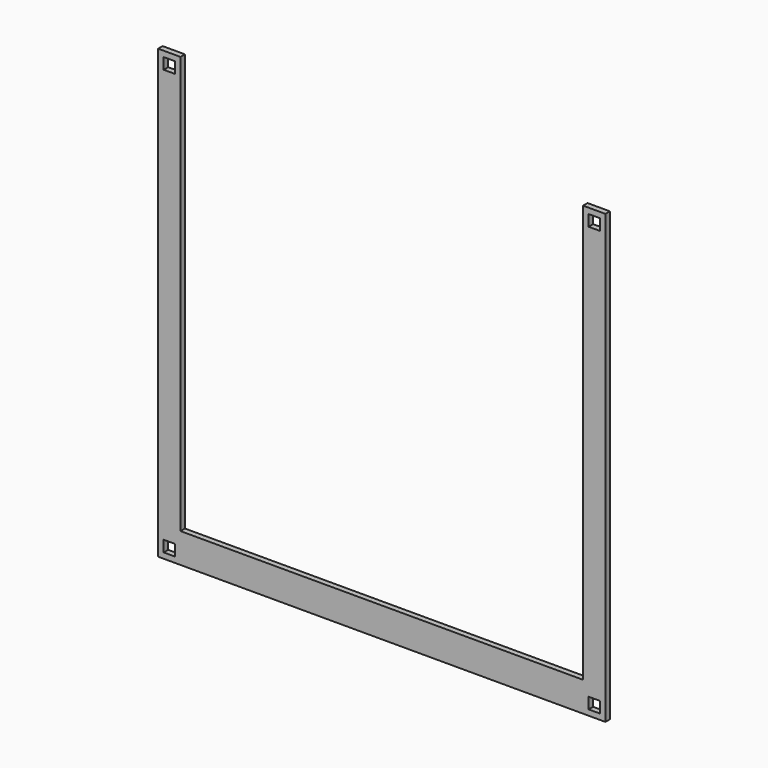
from build123d import *

# Parameters (mm, degrees)
F1_W     = 240
F1_H     = 240
F1_W_2   = 6
F1_H_2   = 6
F1_W_3   = 208
F1_H_3   = 208
F2_DEPTH = 3
F3_DEPTH = 25
F8_W     = 216
F8_H     = 16
F8_W_2   = 208
F8_H_2   = 208
F9_DEPTH = 3.001


with BuildPart() as f2:
    # F1 (on Front) → F2 (new body)
    with BuildSketch(Plane.XZ):
        with Locations((120, 120)):
            Rectangle(F1_W, F1_H)
        with Locations((6, 234)):
            Rectangle(F1_W_2, F1_H_2, mode=Mode.SUBTRACT)
        with Locations((120, 120)):
            Rectangle(F1_W_3, F1_H_3, mode=Mode.SUBTRACT)
        with Locations((6, 234)):
            Rectangle(F1_W_2, F1_H_2)
    extrude(amount=F2_DEPTH)

    # F1 (on Front) → F3 (cut)
    with BuildSketch(Plane.XZ):
        with Locations((6, 234)):
            Rectangle(F1_W_2, F1_H_2)
    extrude(amount=F3_DEPTH, mode=Mode.SUBTRACT)

    # F5: F2 across plane


with BuildPart() as f2_1:
    add(f2.part)
    add(f2.part.mirror(Plane(origin=(120, -1.5, 120), x_dir=(0, -1, 0), z_dir=(-1, 0, 0))), mode=Mode.INTERSECT)

    # F7: F2 across plane


with BuildPart() as f2_2:
    add(f2_1.part)
    add(f2_1.part.mirror(Plane(origin=(120, -1.5, 120), x_dir=(1, 0, 0), z_dir=(0, 0, 1))), mode=Mode.INTERSECT)

    # F8 (on face) → F9 (cut, through all)
    with BuildSketch(Plane.XZ.offset(3)):
        with Locations((120, 248)):
            Rectangle(F8_W, F8_H)
        with Locations((120, 120)):
            Rectangle(F8_W_2, F8_H_2)
        Polygon((228, 240), (12, 240), (12, 16), (16, 16), (16, 224), (224, 224), (224, 16), (228, 16), align=None)
    extrude(amount=-F9_DEPTH, mode=Mode.SUBTRACT)


solid = f2_2.part
